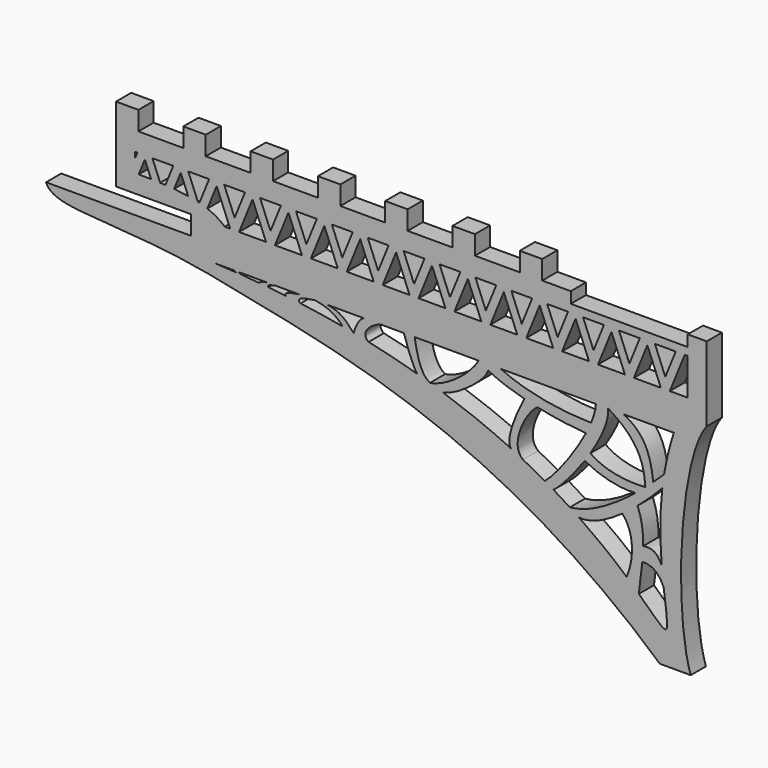
from build123d import *

# Parameters (mm, degrees)
F0_W      = 197.5
F0_H      = 25
F1_DEPTH  = 6.35
F2_W      = 7.5
F2_H      = 6.35
F3_DEPTH  = 6.35
F4_DEPTH  = 2.5
F6_DEPTH  = 6.35
F7_W      = 39.1012286186
F7_H      = 3.7313760072
F8_DEPTH  = 25
F9_DEPTH  = 6.3499999233
F5_W      = 6.35
F5_H      = 6.35
F10_DEPTH = 25


# Not quite as in the source:
# - a length typed as a fraction of an inch, garbled in the dataset ("3 / 203.2 mm" for 3/8 in), is restored
# - a feature names something its author has since deleted; it is built from what else it names


with BuildPart() as f1:
    # F0 (on Front) → F1 (new body)
    with BuildSketch(Plane.XZ):
        with BuildLine():
            add(Edge.make_bspline(
                [(98.75, -5), (89.6041318774, -16.6829489172), (87.6455754042, -62.8589260578), (93.393959105, -80)],
                knots=[0, 0, 0, 0, 75.1910046087, 75.1910046087, 75.1910046087, 75.1910046087], degree=3))
            Line((98.75, -5), (-98.75, -5))
            add(Edge.make_bspline(
                [(-98.75, -5), (-63.6426135898, -22.327804938), (7.773979567, -13.3445840329), (83.1019603317, -80)],
                knots=[0, 0, 0, 0, 196.7107914591, 196.7107914591, 196.7107914591, 196.7107914591], degree=3))
            Line((83.1019603317, -80), (93.393959105, -80))
        make_face()
        with BuildLine():
            add(Edge.make_bspline(
                [(-65.759709787, -10.4816574603), (-63.2453230772, -10.5943254224), (-60.7705862807, -10.7313046439), (-58.3349275577, -10.8914524019)],
                knots=[0, 0, 0, 0, 0.0133310218, 0.0133310218, 0.0133310218, 0.0133310218], degree=3))
            Line((-65.759709787, -10.4816574603), (-58.7879791856, -10.4816574603))
            Line((-58.7879791856, -10.4816574603), (-57.3127828538, -10.4816574603))
            Line((-57.3127828538, -10.4816574603), (-47.9639396071, -10.4816574603))
            Line((-47.9639396071, -10.4816574603), (-45.4429499805, -10.4816574603))
            Line((-45.4429499805, -10.4816574603), (-37.5518873334, -10.4816574603))
            Line((-37.5518873334, -10.4816574603), (-32.1224816144, -10.4816574603))
            Line((-32.1224816144, -10.4816574603), (-28.0221402645, -10.4816574603))
            Line((-28.0221402645, -10.4816574603), (-15.9640572965, -10.4816574603))
            Line((-15.9640572965, -10.4816574603), (-10.2372542024, -10.4816574603))
            Line((-10.2372542024, -10.4816574603), (-2.4892275687, -10.4816574603))
            Line((-2.4892275687, -10.4816574603), (1.1040605605, -10.4816574603))
            Line((1.1040605605, -10.4816574603), (22.4099401385, -10.4816574603))
            Line((22.4099401385, -10.4816574603), (29.8736523837, -10.4816574603))
            Line((29.8736523837, -10.4816574603), (61.6671070457, -10.4816574603))
            Line((61.6671070457, -10.4816574603), (65.7978504896, -10.4816574603))
            Line((65.7978504896, -10.4816574603), (70.9762573242, -10.4816574603))
            Line((70.9762573242, -10.4816574603), (87.7543787006, -10.4816574603))
            add(Edge.make_bspline(
                [(84.48485297, -23.7784693837), (85.1953370139, -19.4532237111), (86.2479291527, -14.9932687844), (87.7543787006, -10.4816574603)],
                knots=[0.9407477342, 0.9407477342, 0.9407477342, 0.9407477342, 1, 1, 1, 1], degree=3))
            add(Edge.make_bspline(
                [(83.8869246499, -28.033053302), (84.0513440433, -26.6316839804), (84.2492959554, -25.212480417), (84.48485297, -23.7784693837)],
                knots=[0.9211029766, 0.9211029766, 0.9211029766, 0.9211029766, 0.9407477342, 0.9407477342, 0.9407477342, 0.9407477342], degree=3))
            add(Edge.make_bspline(
                [(83.6848718472, -50.8613183266), (83.1253506402, -44.3545057691), (82.8910647479, -36.5209055368), (83.8869246499, -28.033053302)],
                knots=[0.8021180686, 0.8021180686, 0.8021180686, 0.8021180686, 0.9211029766, 0.9211029766, 0.9211029766, 0.9211029766], degree=3))
            add(Edge.make_bspline(
                [(84.3356357543, -57.0348066686), (84.1048122326, -55.149453926), (83.8758889834, -53.0827045495), (83.6848718472, -50.8613183266)],
                knots=[0.7614973449, 0.7614973449, 0.7614973449, 0.7614973449, 0.8021180686, 0.8021180686, 0.8021180686, 0.8021180686], degree=3))
            add(Edge.make_bspline(
                [(76.0466038547, -61.7151507236), (81.9550720838, -67.2257504262), (86.8926623373, -72.9460572696), (85.1127651831, -63.38235344), (84.3356357543, -57.0348066686)],
                knots=[0.4567156472, 0.4567156472, 0.4567156472, 0.4567156472, 0.62473676, 0.7614973449, 0.7614973449, 0.7614973449, 0.7614973449], degree=3))
            add(Edge.make_bspline(
                [(71.9460187023, -58.0001276881), (73.4569449838, -59.326355576), (74.8203953797, -60.5715135243), (76.0466038547, -61.7151507236)],
                knots=[0.4218455413, 0.4218455413, 0.4218455413, 0.4218455413, 0.4567156472, 0.4567156472, 0.4567156472, 0.4567156472], degree=3))
            add(Edge.make_bspline(
                [(56.0711816028, -45.7453459696), (62.6000337954, -50.1569782108), (67.8222936938, -54.380494371), (71.9460187023, -58.0001276881)],
                knots=[0.3266756252, 0.3266756252, 0.3266756252, 0.3266756252, 0.4218455413, 0.4218455413, 0.4218455413, 0.4218455413], degree=3))
            add(Edge.make_bspline(
                [(53.0046953922, -43.7233264114), (54.0574936691, -44.4007021836), (55.0794126404, -45.0751944941), (56.0711816028, -45.7453459696)],
                knots=[0.3122187856, 0.3122187856, 0.3122187856, 0.3122187856, 0.3266756252, 0.3266756252, 0.3266756252, 0.3266756252], degree=3))
            add(Edge.make_bspline(
                [(47.5318004772, -40.3497342585), (49.4425367571, -41.4777534857), (51.2657395603, -42.6044733744), (53.0046953922, -43.7233264114)],
                knots=[0.2883397519, 0.2883397519, 0.2883397519, 0.2883397519, 0.3122187856, 0.3122187856, 0.3122187856, 0.3122187856], degree=3))
            add(Edge.make_bspline(
                [(44.6505962547, -38.6863100754), (45.6324034122, -39.2405788357), (46.5926747482, -39.7953134888), (47.5318004772, -40.3497342585)],
                knots=[0.2766032212, 0.2766032212, 0.2766032212, 0.2766032212, 0.2883397519, 0.2883397519, 0.2883397519, 0.2883397519], degree=3))
            add(Edge.make_bspline(
                [(37.3149573755, -34.7702959798), (39.8841702832, -36.066140887), (42.3276605214, -37.3749214801), (44.6505962547, -38.6863100754)],
                knots=[0.2488348287, 0.2488348287, 0.2488348287, 0.2488348287, 0.2766032212, 0.2766032212, 0.2766032212, 0.2766032212], degree=3))
            add(Edge.make_bspline(
                [(33.3332120345, -32.821860666), (34.6928471757, -33.4671703542), (36.0198749712, -34.1170897262), (37.3149573755, -34.7702959798)],
                knots=[0.234837407, 0.234837407, 0.234837407, 0.234837407, 0.2488348287, 0.2488348287, 0.2488348287, 0.2488348287], degree=3))
            add(Edge.make_bspline(
                [(10.4947332364, -23.681362128), (18.9719825925, -26.5045688693), (26.557499928, -29.605973893), (33.3332120345, -32.821860666)],
                knots=[0.165081561, 0.165081561, 0.165081561, 0.165081561, 0.234837407, 0.234837407, 0.234837407, 0.234837407], degree=3))
            add(Edge.make_bspline(
                [(6.2234793397, -22.3067678937), (7.6717739992, -22.7568947859), (9.0954024691, -23.2153383165), (10.4947332364, -23.681362128)],
                knots=[0.1535670358, 0.1535670358, 0.1535670358, 0.1535670358, 0.165081561, 0.165081561, 0.165081561, 0.165081561], degree=3))
            add(Edge.make_bspline(
                [(1.8814823178, -21.0044059123), (3.35287305, -21.4300274782), (4.8000887896, -21.8643811457), (6.2234793397, -22.3067678937)],
                knots=[0.1422505082, 0.1422505082, 0.1422505082, 0.1422505082, 0.1535670358, 0.1535670358, 0.1535670358, 0.1535670358], degree=3))
            add(Edge.make_bspline(
                [(-14.2821822906, -16.9273048212), (-8.5949395005, -18.1623744753), (-3.2118878299, -19.531073146), (1.8814823178, -21.0044059123)],
                knots=[0.1030771858, 0.1030771858, 0.1030771858, 0.1030771858, 0.1422505082, 0.1422505082, 0.1422505082, 0.1422505082], degree=3))
            add(Edge.make_bspline(
                [(-19.2551519245, -15.8974694935), (-17.5722033157, -16.2292806482), (-15.9146611567, -16.5727876707), (-14.2821822906, -16.9273048212)],
                knots=[0.0918327879, 0.0918327879, 0.0918327879, 0.0918327879, 0.1030771858, 0.1030771858, 0.1030771858, 0.1030771858], degree=3))
            add(Edge.make_bspline(
                [(-22.99176564, -15.187903168), (-21.7325254655, -15.4179794431), (-20.4870324208, -15.6545911977), (-19.2551519245, -15.8974694935)],
                knots=[0.0836021417, 0.0836021417, 0.0836021417, 0.0836021417, 0.0918327879, 0.0918327879, 0.0918327879, 0.0918327879], degree=3))
            add(Edge.make_bspline(
                [(-37.0301090074, -12.9832383793), (-32.170871054, -13.6264103929), (-27.4934728723, -14.365394442), (-22.99176564, -15.187903168)],
                knots=[0.0541780811, 0.0541780811, 0.0541780811, 0.0541780811, 0.0836021417, 0.0836021417, 0.0836021417, 0.0836021417], degree=3))
            add(Edge.make_bspline(
                [(-41.8800378972, -12.3806058964), (-40.2436101899, -12.5708446493), (-38.6270399752, -12.7718675191), (-37.0301090074, -12.9832383793)],
                knots=[0.0445082122, 0.0445082122, 0.0445082122, 0.0445082122, 0.0541780811, 0.0541780811, 0.0541780811, 0.0541780811], degree=3))
            add(Edge.make_bspline(
                [(-47.8362962746, -11.7451335191), (-45.8222313414, -11.9410389088), (-43.8369362876, -12.1531116371), (-41.8800378972, -12.3806058964)],
                knots=[0.0329446395, 0.0329446395, 0.0329446395, 0.0329446395, 0.0445082122, 0.0445082122, 0.0445082122, 0.0445082122], degree=3))
            add(Edge.make_bspline(
                [(-50.9760160676, -11.4549833836), (-49.9217537521, -11.5473301551), (-48.875197562, -11.6440809868), (-47.8362962746, -11.7451335191)],
                knots=[0.0269798812, 0.0269798812, 0.0269798812, 0.0269798812, 0.0329446395, 0.0329446395, 0.0329446395, 0.0329446395], degree=3))
            add(Edge.make_bspline(
                [(-55.2391494684, -11.108963422), (-53.8042929939, -11.2162939437), (-52.3832891368, -11.3317150824), (-50.9760160676, -11.4549833836)],
                knots=[0.0190178744, 0.0190178744, 0.0190178744, 0.0190178744, 0.0269798812, 0.0269798812, 0.0269798812, 0.0269798812], degree=3))
            add(Edge.make_bspline(
                [(-58.3349275577, -10.8914524019), (-57.2959050051, -10.9597694986), (-56.2639937725, -11.0323027415), (-55.2391494684, -11.108963422)],
                knots=[0.0133310218, 0.0133310218, 0.0133310218, 0.0133310218, 0.0190178744, 0.0190178744, 0.0190178744, 0.0190178744], degree=3))
        make_face(mode=Mode.SUBTRACT)
        with Locations((0, 7.5)):
            Rectangle(F0_W, F0_H)
        Polygon((92.4, 13.65), (92.4, 1.35), (86.4, 1.35), (83.4, 1.35), (74.4, 1.35), (71.4, 1.35), (62.4, 1.35), (59.4, 1.35), (50.4, 1.35), (47.4, 1.35), (38.4, 1.35), (35.4, 1.35), (26.4, 1.35), (23.4, 1.35), (14.4, 1.35), (11.4, 1.35), (2.4, 1.35), (-0.6, 1.35), (-9.6, 1.35), (-12.6, 1.35), (-21.6, 1.35), (-24.6, 1.35), (-33.6, 1.35), (-36.6, 1.35), (-45.6, 1.35), (-48.6, 1.35), (-57.6, 1.35), (-60.6, 1.35), (-62.4, 1.35), (-69.6, 1.35), (-72.6, 1.35), (-81.6, 1.35), (-84.6, 1.35), (-92.4, 1.35), (-92.4, 4.31), (-92.4, 7.35), (-92.4, 11.71), (-92.4, 13.65), (-91.6135135135, 13.65), (-90.6, 16.15), (-89.5864864865, 13.65), (-88.6135135135, 13.65), (-87.6, 16.15), (-86.5864864865, 13.65), (-79.6135135135, 13.65), (-78.6, 16.15), (-77.5864864865, 13.65), (-76.6135135135, 13.65), (-75.6, 16.15), (-74.5864864865, 13.65), (-67.6135135135, 13.65), (-66.6, 16.15), (-65.5864864865, 13.65), (-64.6135135135, 13.65), (-63.6, 16.15), (-62.5864864865, 13.65), (-55.6135135135, 13.65), (-54.6, 16.15), (-53.5864864865, 13.65), (-52.6135135135, 13.65), (-51.6, 16.15), (-50.5864864865, 13.65), (-43.6135135135, 13.65), (-42.6, 16.15), (-41.5864864865, 13.65), (-40.6135135135, 13.65), (-39.6, 16.15), (-38.5864864865, 13.65), (-31.6135135135, 13.65), (-30.6, 16.15), (-29.5864864865, 13.65), (-28.6135135135, 13.65), (-27.6, 16.15), (-26.5864864865, 13.65), (-19.6135135135, 13.65), (-18.6, 16.15), (-17.5864864865, 13.65), (-16.6135135135, 13.65), (-15.6, 16.15), (-14.5864864865, 13.65), (-7.6135135135, 13.65), (-6.6, 16.15), (-5.5864864865, 13.65), (-4.6135135135, 13.65), (-3.6, 16.15), (-2.5864864865, 13.65), (4.3864864865, 13.65), (5.4, 16.15), (6.4135135135, 13.65), (7.3864864865, 13.65), (8.4, 16.15), (9.4135135135, 13.65), (16.3864864865, 13.65), (17.4, 16.15), (18.4135135135, 13.65), (19.3864864865, 13.65), (20.4, 16.15), (21.4135135135, 13.65), (28.3864864865, 13.65), (29.4, 16.15), (30.4135135135, 13.65), (31.3864864865, 13.65), (32.4, 16.15), (33.4135135135, 13.65), (40.3864864865, 13.65), (41.4, 16.15), (42.4135135135, 13.65), (43.3864864865, 13.65), (44.4, 16.15), (45.4135135135, 13.65), (52.3864864865, 13.65), (53.4, 16.15), (54.4135135135, 13.65), (55.3864864865, 13.65), (56.4, 16.15), (57.4135135135, 13.65), (64.3864864865, 13.65), (65.4, 16.15), (66.4135135135, 13.65), (67.3864864865, 13.65), (68.4, 16.15), (69.4135135135, 13.65), (76.3864864865, 13.65), (77.4, 16.15), (78.4135135135, 13.65), (79.3864864865, 13.65), (80.4, 16.15), (81.4135135135, 13.65), (88.3864864865, 13.65), (91.3864864865, 13.65), align=None, mode=Mode.SUBTRACT)
        with BuildLine():
            Line((65.7978504896, -10.4816574603), (61.6671070457, -10.4816574603))
            add(Edge.make_bspline(
                [(60.0847187439, -16.5496386622), (61.0756793988, -14.2032740615), (61.6736950942, -12.0951756308), (61.6671070457, -10.4816574603)],
                knots=[25.462285853, 25.462285853, 25.462285853, 25.462285853, 32.9403106943, 32.9403106943, 32.9403106943, 32.9403106943], degree=3))
            add(Edge.make_bspline(
                [(58.3588024867, -20.1612836249), (59.0126430275, -18.9199905731), (59.5963911144, -17.7058850356), (60.0847187439, -16.5496386622)],
                knots=[21.7772493925, 21.7772493925, 21.7772493925, 21.7772493925, 25.462285853, 25.462285853, 25.462285853, 25.462285853], degree=3))
            add(Edge.make_bspline(
                [(44.6505962547, -38.6863100754), (48.1829739645, -35.7819743058), (54.4948384056, -27.4968822406), (58.3588024867, -20.1612836249)],
                knots=[0, 0, 0, 0, 21.7772493925, 21.7772493925, 21.7772493925, 21.7772493925], degree=3))
            add(Edge.make_bspline(
                [(44.6505962547, -38.6863100754), (45.6324034122, -39.2405788357), (46.5926747482, -39.7953134888), (47.5318004772, -40.3497342585)],
                knots=[0.2766032212, 0.2766032212, 0.2766032212, 0.2766032212, 0.2883397519, 0.2883397519, 0.2883397519, 0.2883397519], degree=3))
            add(Edge.make_bspline(
                [(57.9517171021, -28.4242599565), (54.3108044366, -33.6350813387), (50.2093884078, -38.282844387), (47.5318004772, -40.3497342585)],
                knots=[19.2539293083, 19.2539293083, 19.2539293083, 19.2539293083, 35.0107211391, 35.0107211391, 35.0107211391, 35.0107211391], degree=3))
            add(Edge.make_bspline(
                [(59.8575436042, -25.5745284736), (59.2443879934, -26.5348050429), (58.6054762028, -27.4886094167), (57.9517171021, -28.4242599565)],
                knots=[16.4246535187, 16.4246535187, 16.4246535187, 16.4246535187, 19.2539293083, 19.2539293083, 19.2539293083, 19.2539293083], degree=3))
            add(Edge.make_bspline(
                [(65.7978504896, -10.4816574603), (66.1085797514, -14.2071182078), (63.4170652659, -19.9998828383), (59.8575436042, -25.5745284736)],
                knots=[0, 0, 0, 0, 16.4246535187, 16.4246535187, 16.4246535187, 16.4246535187], degree=3))
        make_face()
        with BuildLine():
            Line((29.8736523837, -10.4816574603), (22.4099401385, -10.4816574603))
            add(Edge.make_bspline(
                [(25.6780489338, -12.3534352143), (24.4977620539, -11.7616059964), (23.4022584509, -11.1376377151), (22.4099401385, -10.4816574603)],
                knots=[32.7980602328, 32.7980602328, 32.7980602328, 32.7980602328, 37.2292340348, 37.2292340348, 37.2292340348, 37.2292340348], degree=3))
            add(Edge.make_bspline(
                [(37.7584589003, -16.7207107112), (33.3129817339, -15.5423673153), (29.1324045595, -14.0855468079), (25.6780489338, -12.3534352143)],
                knots=[19.8293062687, 19.8293062687, 19.8293062687, 19.8293062687, 32.7980602328, 32.7980602328, 32.7980602328, 32.7980602328], degree=3))
            add(Edge.make_bspline(
                [(42.1803625343, -17.7854881771), (40.6888661107, -17.4603079049), (39.2095499868, -17.1053451464), (37.7584589003, -16.7207107112)],
                knots=[15.5960501804, 15.5960501804, 15.5960501804, 15.5960501804, 19.8293062687, 19.8293062687, 19.8293062687, 19.8293062687], degree=3))
            add(Edge.make_bspline(
                [(58.3588024867, -20.1612836249), (53.3355507823, -19.7772875995), (47.6752942326, -18.9835087403), (42.1803625343, -17.7854881771)],
                knots=[0, 0, 0, 0, 15.5960501804, 15.5960501804, 15.5960501804, 15.5960501804], degree=3))
            add(Edge.make_bspline(
                [(58.3588024867, -20.1612836249), (59.0126430275, -18.9199905731), (59.5963911144, -17.7058850356), (60.0847187439, -16.5496386622)],
                knots=[21.7772493925, 21.7772493925, 21.7772493925, 21.7772493925, 25.462285853, 25.462285853, 25.462285853, 25.462285853], degree=3))
            add(Edge.make_bspline(
                [(60.0847187439, -16.5496386622), (47.3331118165, -16.3230231964), (36.7021560669, -13.6903477833), (29.8736523837, -10.4816574603)],
                knots=[0, 0, 0, 0, 30.8144272458, 30.8144272458, 30.8144272458, 30.8144272458], degree=3))
        make_face()
        with BuildLine():
            add(Edge.make_bspline(
                [(78.2400502629, -29.5795594501), (79.162668759, -28.7799506841), (80.0339477004, -28.0008363248), (80.84262329, -27.2596680265)],
                knots=[27.3886664947, 27.3886664947, 27.3886664947, 27.3886664947, 30.9554664602, 30.9554664602, 30.9554664602, 30.9554664602], degree=3))
            add(Edge.make_bspline(
                [(74.8700098337, -32.3933389933), (76.0498454996, -31.4460030072), (77.1789047527, -30.4992258728), (78.2400502629, -29.5795594501)],
                knots=[23.2863275706, 23.2863275706, 23.2863275706, 23.2863275706, 27.3886664947, 27.3886664947, 27.3886664947, 27.3886664947], degree=3))
            add(Edge.make_bspline(
                [(53.0046953922, -43.7233264114), (59.8396137806, -43.1661743955), (68.1728450446, -37.7707533169), (74.8700098337, -32.3933389933)],
                knots=[0, 0, 0, 0, 23.2863275706, 23.2863275706, 23.2863275706, 23.2863275706], degree=3))
            add(Edge.make_bspline(
                [(53.0046953922, -43.7233264114), (54.0574936691, -44.4007021836), (55.0794126404, -45.0751944941), (56.0711816028, -45.7453459696)],
                knots=[0.3122187856, 0.3122187856, 0.3122187856, 0.3122187856, 0.3266756252, 0.3266756252, 0.3266756252, 0.3266756252], degree=3))
            add(Edge.make_bspline(
                [(56.0711816028, -45.7453459696), (60.2977500573, -46.1208300554), (65.6205880142, -43.3719518378), (70.5272099637, -39.8740143131)],
                knots=[0, 0, 0, 0, 14.8454914625, 14.8454914625, 14.8454914625, 14.8454914625], degree=3))
            add(Edge.make_bspline(
                [(70.5272099637, -39.8740143131), (72.30613066, -38.6058193063), (74.0303413505, -37.2391633124), (75.6277622982, -35.8872449137)],
                knots=[14.8454914625, 14.8454914625, 14.8454914625, 14.8454914625, 20.2277997552, 20.2277997552, 20.2277997552, 20.2277997552], degree=3))
            add(Edge.make_bspline(
                [(75.6277622982, -35.8872449137), (79.4114234149, -32.68508265), (82.4837566461, -29.5656026462), (83.8869246499, -28.033053302)],
                knots=[20.2277997552, 20.2277997552, 20.2277997552, 20.2277997552, 32.9763683993, 32.9763683993, 32.9763683993, 32.9763683993], degree=3))
            add(Edge.make_bspline(
                [(83.8869246499, -28.033053302), (84.0513440433, -26.6316839804), (84.2492959554, -25.212480417), (84.48485297, -23.7784693837)],
                knots=[0.9211029766, 0.9211029766, 0.9211029766, 0.9211029766, 0.9407477342, 0.9407477342, 0.9407477342, 0.9407477342], degree=3))
            add(Edge.make_bspline(
                [(80.84262329, -27.2596680265), (82.2734968467, -25.9482421187), (83.5083724964, -24.7556173344), (84.48485297, -23.7784693837)],
                knots=[30.9554664602, 30.9554664602, 30.9554664602, 30.9554664602, 37.2665754125, 37.2665754125, 37.2665754125, 37.2665754125], degree=3))
        make_face()
        with BuildLine():
            add(Edge.make_bspline(
                [(70.5272099637, -39.8740143131), (74.9861299992, -44.78995502), (74.1921216249, -53.1270802021), (71.9460187023, -58.0001276881)],
                knots=[0, 0, 0, 0, 18.1815567078, 18.1815567078, 18.1815567078, 18.1815567078], degree=3))
            add(Edge.make_bspline(
                [(71.9460187023, -58.0001276881), (73.4569449838, -59.326355576), (74.8203953797, -60.5715135243), (76.0466038547, -61.7151507236)],
                knots=[0.4218455413, 0.4218455413, 0.4218455413, 0.4218455413, 0.4567156472, 0.4567156472, 0.4567156472, 0.4567156472], degree=3))
            add(Edge.make_bspline(
                [(77.2107662738, -51.8775882795), (76.8736521354, -55.2196716314), (76.3424581234, -58.5197961174), (76.0466038547, -61.7151507236)],
                knots=[15.8511875894, 15.8511875894, 15.8511875894, 15.8511875894, 25.8313016856, 25.8313016856, 25.8313016856, 25.8313016856], degree=3))
            add(Edge.make_bspline(
                [(77.5129660357, -47.1400606018), (77.4849713904, -48.7241622392), (77.3693402282, -50.3055172421), (77.2107662738, -51.8775882795)],
                knots=[11.1566762117, 11.1566762117, 11.1566762117, 11.1566762117, 15.8511875894, 15.8511875894, 15.8511875894, 15.8511875894], degree=3))
            add(Edge.make_bspline(
                [(75.6277622982, -35.8872449137), (77.1510621988, -39.5951980588), (77.5794963236, -43.3753857223), (77.5129660357, -47.1400606018)],
                knots=[0, 0, 0, 0, 11.1566762117, 11.1566762117, 11.1566762117, 11.1566762117], degree=3))
            add(Edge.make_bspline(
                [(70.5272099637, -39.8740143131), (72.30613066, -38.6058193063), (74.0303413505, -37.2391633124), (75.6277622982, -35.8872449137)],
                knots=[14.8454914625, 14.8454914625, 14.8454914625, 14.8454914625, 20.2277997552, 20.2277997552, 20.2277997552, 20.2277997552], degree=3))
        make_face()
        with BuildLine():
            Line((70.9762573242, -10.4816574603), (65.7978504896, -10.4816574603))
            add(Edge.make_bspline(
                [(78.2400502629, -29.5795594501), (77.7780916973, -21.8921517618), (75.1671940088, -16.122511588), (65.7978504896, -10.4816574603)],
                knots=[0, 0, 0, 0, 22.7933805217, 22.7933805217, 22.7933805217, 22.7933805217], degree=3))
            add(Edge.make_bspline(
                [(78.2400502629, -29.5795594501), (79.162668759, -28.7799506841), (80.0339477004, -28.0008363248), (80.84262329, -27.2596680265)],
                knots=[27.3886664947, 27.3886664947, 27.3886664947, 27.3886664947, 30.9554664602, 30.9554664602, 30.9554664602, 30.9554664602], degree=3))
            add(Edge.make_bspline(
                [(80.84262329, -27.2596680265), (80.1640096856, -20.6172912009), (78.5020440817, -14.1374813393), (70.9762573242, -10.4816574603)],
                knots=[0, 0, 0, 0, 19.4639876677, 19.4639876677, 19.4639876677, 19.4639876677], degree=3))
        make_face()
        with BuildLine():
            add(Edge.make_bspline(
                [(22.4099401385, -10.4816574603), (20.5344334245, -14.4370757043), (12.4321363532, -21.3281778624), (6.2234793397, -22.3067678937)],
                knots=[0, 0, 0, 0, 20.0458162705, 20.0458162705, 20.0458162705, 20.0458162705], degree=3))
            add(Edge.make_bspline(
                [(6.2234793397, -22.3067678937), (7.6717739992, -22.7568947859), (9.0954024691, -23.2153383165), (10.4947332364, -23.681362128)],
                knots=[0.1535670358, 0.1535670358, 0.1535670358, 0.1535670358, 0.165081561, 0.165081561, 0.165081561, 0.165081561], degree=3))
            add(Edge.make_bspline(
                [(25.6780489338, -12.3534352143), (24.5176322607, -16.0640382603), (15.1727138842, -23.0167808315), (10.4947332364, -23.681362128)],
                knots=[0, 0, 0, 0, 18.9434686298, 18.9434686298, 18.9434686298, 18.9434686298], degree=3))
            add(Edge.make_bspline(
                [(25.6780489338, -12.3534352143), (24.4977620539, -11.7616059964), (23.4022584509, -11.1376377151), (22.4099401385, -10.4816574603)],
                knots=[32.7980602328, 32.7980602328, 32.7980602328, 32.7980602328, 37.2292340348, 37.2292340348, 37.2292340348, 37.2292340348], degree=3))
        make_face()
        with BuildLine():
            add(Edge.make_bspline(
                [(74.8700098337, -32.3933389933), (76.0498454996, -31.4460030072), (77.1789047527, -30.4992258728), (78.2400502629, -29.5795594501)],
                knots=[23.2863275706, 23.2863275706, 23.2863275706, 23.2863275706, 27.3886664947, 27.3886664947, 27.3886664947, 27.3886664947], degree=3))
            add(Edge.make_bspline(
                [(59.8575436042, -25.5745284736), (64.3577575684, -28.8347955793), (71.3215619326, -30.0623122603), (78.2400502629, -29.5795594501)],
                knots=[0, 0, 0, 0, 18.8137403027, 18.8137403027, 18.8137403027, 18.8137403027], degree=3))
            add(Edge.make_bspline(
                [(59.8575436042, -25.5745284736), (59.2443879934, -26.5348050429), (58.6054762028, -27.4886094167), (57.9517171021, -28.4242599565)],
                knots=[16.4246535187, 16.4246535187, 16.4246535187, 16.4246535187, 19.2539293083, 19.2539293083, 19.2539293083, 19.2539293083], degree=3))
            add(Edge.make_bspline(
                [(57.9517171021, -28.4242599565), (61.9971491396, -30.5344350636), (68.0639222264, -32.7770151198), (74.8700098337, -32.3933389933)],
                knots=[0, 0, 0, 0, 17.3776355513, 17.3776355513, 17.3776355513, 17.3776355513], degree=3))
        make_face()
        with BuildLine():
            add(Edge.make_bspline(
                [(37.7584589003, -16.7207107112), (36.0090921977, -19.8501714013), (31.0873150466, -30.4321467039), (33.3332120345, -32.821860666)],
                knots=[0, 0, 0, 0, 16.698198696, 16.698198696, 16.698198696, 16.698198696], degree=3))
            add(Edge.make_bspline(
                [(33.3332120345, -32.821860666), (34.6928471757, -33.4671703542), (36.0198749712, -34.1170897262), (37.3149573755, -34.7702959798)],
                knots=[0.234837407, 0.234837407, 0.234837407, 0.234837407, 0.2488348287, 0.2488348287, 0.2488348287, 0.2488348287], degree=3))
            add(Edge.make_bspline(
                [(42.1803625343, -17.7854881771), (38.6197759533, -20.0084939689), (32.4902777722, -31.0945309624), (37.3149573755, -34.7702959798)],
                knots=[0, 0, 0, 0, 17.667933197, 17.667933197, 17.667933197, 17.667933197], degree=3))
            add(Edge.make_bspline(
                [(42.1803625343, -17.7854881771), (40.6888661107, -17.4603079049), (39.2095499868, -17.1053451464), (37.7584589003, -16.7207107112)],
                knots=[15.5960501804, 15.5960501804, 15.5960501804, 15.5960501804, 19.8293062687, 19.8293062687, 19.8293062687, 19.8293062687], degree=3))
        make_face()
        with BuildLine():
            Line((-92.4, 1.35), (-84.6, 1.35))
            Line((-84.6, 1.35), (-87.0299326713, 7.3438339226))
            add(Edge.make_bspline(
                [(-91.1623099358, 7.362968825), (-89.7087542708, 7.3735352095), (-88.3329530456, 7.3667226405), (-87.0299326713, 7.3438339226)],
                knots=[0.6111811792, 0.6111811792, 0.6111811792, 0.6111811792, 2.7969142011, 2.7969142011, 2.7969142011, 2.7969142011], degree=3))
            Line((-91.1623099358, 7.362968825), (-92.4, 4.31))
            Line((-92.4, 4.31), (-92.4, 1.35))
        make_face()
        with BuildLine():
            Line((-81.6, 1.35), (-72.6, 1.35))
            Line((-72.6, 1.35), (-74.6445363191, 6.3931895871))
            add(Edge.make_bspline(
                [(-79.3242019839, 6.9636351063), (-77.5879288026, 6.8107230955), (-76.0366566301, 6.6183175745), (-74.6445363191, 6.3931895871)],
                knots=[7.685023711, 7.685023711, 7.685023711, 7.685023711, 11.4710988351, 11.4710988351, 11.4710988351, 11.4710988351], degree=3))
            Line((-79.3242019839, 6.9636351063), (-81.6, 1.35))
        make_face()
        with BuildLine():
            add(Edge.make_bspline(
                [(84.3356357543, -57.0348066686), (84.1048122326, -55.149453926), (83.8758889834, -53.0827045495), (83.6848718472, -50.8613183266)],
                knots=[0.7614973449, 0.7614973449, 0.7614973449, 0.7614973449, 0.8021180686, 0.8021180686, 0.8021180686, 0.8021180686], degree=3))
            add(Edge.make_bspline(
                [(77.5129660357, -47.1400606018), (81.1000242829, -46.5764813125), (82.4895426631, -48.2439063489), (83.6848718472, -50.8613183266)],
                knots=[0, 0, 0, 0, 7.2069536144, 7.2069536144, 7.2069536144, 7.2069536144], degree=3))
            add(Edge.make_bspline(
                [(77.5129660357, -47.1400606018), (77.4849713904, -48.7241622392), (77.3693402282, -50.3055172421), (77.2107662738, -51.8775882795)],
                knots=[11.1566762117, 11.1566762117, 11.1566762117, 11.1566762117, 15.8511875894, 15.8511875894, 15.8511875894, 15.8511875894], degree=3))
            add(Edge.make_bspline(
                [(77.2107662738, -51.8775882795), (79.8296034336, -51.8566630781), (82.2116434574, -52.5315739214), (84.3356357543, -57.0348066686)],
                knots=[0, 0, 0, 0, 8.795491267, 8.795491267, 8.795491267, 8.795491267], degree=3))
        make_face()
        with BuildLine():
            Line((1.1040605605, -10.4816574603), (-2.4892275687, -10.4816574603))
            add(Edge.make_bspline(
                [(-2.4892275687, -10.4816574603), (-1.5305990819, -13.7633346021), (0.383801406, -18.9892837864), (1.8814823178, -21.0044059123)],
                knots=[0, 0, 0, 0, 11.3943556156, 11.3943556156, 11.3943556156, 11.3943556156], degree=3))
            add(Edge.make_bspline(
                [(1.8814823178, -21.0044059123), (3.35287305, -21.4300274782), (4.8000887896, -21.8643811457), (6.2234793397, -22.3067678937)],
                knots=[0.1422505082, 0.1422505082, 0.1422505082, 0.1422505082, 0.1535670358, 0.1535670358, 0.1535670358, 0.1535670358], degree=3))
            add(Edge.make_bspline(
                [(6.2234793397, -22.3067678937), (2.6628852488, -20.4860014846), (1.6135276528, -13.426464051), (1.1040605605, -10.4816574603)],
                knots=[0, 0, 0, 0, 12.8857163324, 12.8857163324, 12.8857163324, 12.8857163324], degree=3))
        make_face()
        with BuildLine():
            Line((-10.2372542024, -10.4816574603), (-15.9640572965, -10.4816574603))
            add(Edge.make_bspline(
                [(-15.9640572965, -10.4816574603), (-17.7565403283, -11.405239813), (-19.0194105432, -14.6001277884), (-19.2551519245, -15.8974694935)],
                knots=[0, 0, 0, 0, 6.3373751529, 6.3373751529, 6.3373751529, 6.3373751529], degree=3))
            add(Edge.make_bspline(
                [(-19.2551519245, -15.8974694935), (-17.5722033157, -16.2292806482), (-15.9146611567, -16.5727876707), (-14.2821822906, -16.9273048212)],
                knots=[0.0918327879, 0.0918327879, 0.0918327879, 0.0918327879, 0.1030771858, 0.1030771858, 0.1030771858, 0.1030771858], degree=3))
            add(Edge.make_bspline(
                [(-10.2372542024, -10.4816574603), (-14.8369930685, -11.9666904211), (-16.7967783765, -15.3098717261), (-14.2821822906, -16.9273048212)],
                knots=[0, 0, 0, 0, 7.6097183351, 7.6097183351, 7.6097183351, 7.6097183351], degree=3))
        make_face()
        with BuildLine():
            Line((-28.0221402645, -10.4816574603), (-32.1224816144, -10.4816574603))
            add(Edge.make_bspline(
                [(-32.1224816144, -10.4816574603), (-26.3739395887, -11.374656111), (-24.0345019539, -13.9484412274), (-22.99176564, -15.187903168)],
                knots=[0, 0, 0, 0, 10.2722306665, 10.2722306665, 10.2722306665, 10.2722306665], degree=3))
            add(Edge.make_bspline(
                [(-22.99176564, -15.187903168), (-21.7325254655, -15.4179794431), (-20.4870324208, -15.6545911977), (-19.2551519245, -15.8974694935)],
                knots=[0.0836021417, 0.0836021417, 0.0836021417, 0.0836021417, 0.0918327879, 0.0918327879, 0.0918327879, 0.0918327879], degree=3))
            add(Edge.make_bspline(
                [(-19.2551519245, -15.8974694935), (-21.3651643768, -14.2235838269), (-22.4346164614, -11.307887733), (-28.0221402645, -10.4816574603)],
                knots=[0, 0, 0, 0, 10.3049068183, 10.3049068183, 10.3049068183, 10.3049068183], degree=3))
        make_face()
        with BuildLine():
            Line((-69.6, 1.35), (-62.4, 1.35))
            add(Edge.make_bspline(
                [(-68.2077429312, 4.784234103), (-65.461468977, 3.7637652405), (-63.7904450742, 2.5496339353), (-62.4, 1.35)],
                knots=[18.7336175286, 18.7336175286, 18.7336175286, 18.7336175286, 30.5941170816, 30.5941170816, 30.5941170816, 30.5941170816], degree=3))
            Line((-68.2077429312, 4.784234103), (-69.6, 1.35))
        make_face()
        with BuildLine():
            Line((-87.0299326713, 7.3438339226), (-84.6, 1.35))
            Line((-84.6, 1.35), (-83.1, 5.05))
            Line((-83.1, 5.05), (-83.9946804025, 7.2568783261))
            add(Edge.make_bspline(
                [(-87.0299326713, 7.3438339226), (-85.9710046553, 7.3252329052), (-84.9601437029, 7.296014627), (-83.9946804025, 7.2568783261)],
                knots=[2.7969142011, 2.7969142011, 2.7969142011, 2.7969142011, 4.573197963, 4.573197963, 4.573197963, 4.573197963], degree=3))
        make_face()
        with BuildLine():
            Line((-83.1, 5.05), (-81.6, 1.35))
            Line((-81.6, 1.35), (-79.3242019839, 6.9636351063))
            add(Edge.make_bspline(
                [(-82.2396503054, 7.1721959134), (-81.2134817801, 7.1144023953), (-80.2429422559, 7.0445477323), (-79.3242019839, 6.9636351063)],
                knots=[5.6816409906, 5.6816409906, 5.6816409906, 5.6816409906, 7.685023711, 7.685023711, 7.685023711, 7.685023711], degree=3))
            Line((-82.2396503054, 7.1721959134), (-83.1, 5.05))
        make_face()
        with BuildLine():
            Line((-32.1224816144, -10.4816574603), (-37.5518873334, -10.4816574603))
            add(Edge.make_bspline(
                [(-37.5518873334, -10.4816574603), (-39.5294241607, -10.7246097177), (-43.3542957133, -11.6059756945), (-41.8800378972, -12.3806058964)],
                knots=[0, 0, 0, 0, 4.7264037562, 4.7264037562, 4.7264037562, 4.7264037562], degree=3))
            add(Edge.make_bspline(
                [(-41.8800378972, -12.3806058964), (-40.2436101899, -12.5708446493), (-38.6270399752, -12.7718675191), (-37.0301090074, -12.9832383793)],
                knots=[0.0445082122, 0.0445082122, 0.0445082122, 0.0445082122, 0.0541780811, 0.0541780811, 0.0541780811, 0.0541780811], degree=3))
            add(Edge.make_bspline(
                [(-32.1224816144, -10.4816574603), (-37.0871126652, -11.0053345561), (-38.6487748038, -12.0604483888), (-37.0301090074, -12.9832383793)],
                knots=[0, 0, 0, 0, 5.5084220719, 5.5084220719, 5.5084220719, 5.5084220719], degree=3))
        make_face()
        with BuildLine():
            Line((-74.6445363191, 6.3931895871), (-72.6, 1.35))
            Line((-72.6, 1.35), (-71.1, 5.05))
            Line((-71.1, 5.05), (-71.3804824815, 5.7418567877))
            add(Edge.make_bspline(
                [(-74.6445363191, 6.3931895871), (-73.4436123593, 6.1989810895), (-72.3611258914, 5.9804212158), (-71.3804824815, 5.7418567877)],
                knots=[11.4710988351, 11.4710988351, 11.4710988351, 11.4710988351, 14.7371874729, 14.7371874729, 14.7371874729, 14.7371874729], degree=3))
        make_face()
        with BuildLine():
            Line((-71.1, 5.05), (-69.6, 1.35))
            Line((-69.6, 1.35), (-68.2077429312, 4.784234103))
            add(Edge.make_bspline(
                [(-70.8713985904, 5.6138834771), (-69.8813559343, 5.3567733844), (-68.9998261767, 5.0785588143), (-68.2077429312, 4.784234103)],
                knots=[15.3127996729, 15.3127996729, 15.3127996729, 15.3127996729, 18.7336175286, 18.7336175286, 18.7336175286, 18.7336175286], degree=3))
            Line((-70.8713985904, 5.6138834771), (-71.1, 5.05))
        make_face()
        Polygon((-84.6, 1.35), (-81.6, 1.35), (-83.1, 5.05), align=None)
        Polygon((-72.6, 1.35), (-69.6, 1.35), (-71.1, 5.05), align=None)
        with BuildLine():
            Line((-45.4429499805, -10.4816574603), (-47.9639396071, -10.4816574603))
            add(Edge.make_bspline(
                [(-47.9639396071, -10.4816574603), (-49.7504658997, -10.6397052337), (-50.426291577, -11.0352661865), (-50.9760160676, -11.4549833836)],
                knots=[0, 0, 0, 0, 3.1654332968, 3.1654332968, 3.1654332968, 3.1654332968], degree=3))
            add(Edge.make_bspline(
                [(-50.9760160676, -11.4549833836), (-49.9217537521, -11.5473301551), (-48.875197562, -11.6440809868), (-47.8362962746, -11.7451335191)],
                knots=[0.0269798812, 0.0269798812, 0.0269798812, 0.0269798812, 0.0329446395, 0.0329446395, 0.0329446395, 0.0329446395], degree=3))
            add(Edge.make_bspline(
                [(-45.4429499805, -10.4816574603), (-47.6661846042, -10.8779086773), (-48.3162734611, -11.3382417703), (-47.8362962746, -11.7451335191)],
                knots=[0, 0, 0, 0, 2.7063773267, 2.7063773267, 2.7063773267, 2.7063773267], degree=3))
        make_face()
        Polygon((76.3864864865, 13.65), (78.4135135135, 13.65), (77.4, 16.15), align=None)
        Polygon((79.3864864865, 13.65), (81.4135135135, 13.65), (80.4, 16.15), align=None)
        Polygon((-88.6135135135, 13.65), (-86.5864864865, 13.65), (-87.6, 16.15), align=None)
        Polygon((-91.6135135135, 13.65), (-89.5864864865, 13.65), (-90.6, 16.15), align=None)
        Polygon((-79.6135135135, 13.65), (-77.5864864865, 13.65), (-78.6, 16.15), align=None)
        Polygon((-76.6135135135, 13.65), (-74.5864864865, 13.65), (-75.6, 16.15), align=None)
        Polygon((-67.6135135135, 13.65), (-65.5864864865, 13.65), (-66.6, 16.15), align=None)
        Polygon((-64.6135135135, 13.65), (-62.5864864865, 13.65), (-63.6, 16.15), align=None)
        Polygon((-55.6135135135, 13.65), (-53.5864864865, 13.65), (-54.6, 16.15), align=None)
        Polygon((-52.6135135135, 13.65), (-50.5864864865, 13.65), (-51.6, 16.15), align=None)
        Polygon((-43.6135135135, 13.65), (-41.5864864865, 13.65), (-42.6, 16.15), align=None)
        Polygon((-40.6135135135, 13.65), (-38.5864864865, 13.65), (-39.6, 16.15), align=None)
        Polygon((-31.6135135135, 13.65), (-29.5864864865, 13.65), (-30.6, 16.15), align=None)
        Polygon((-28.6135135135, 13.65), (-26.5864864865, 13.65), (-27.6, 16.15), align=None)
        Polygon((-19.6135135135, 13.65), (-17.5864864865, 13.65), (-18.6, 16.15), align=None)
        Polygon((-16.6135135135, 13.65), (-14.5864864865, 13.65), (-15.6, 16.15), align=None)
        Polygon((-7.6135135135, 13.65), (-5.5864864865, 13.65), (-6.6, 16.15), align=None)
        Polygon((-4.6135135135, 13.65), (-2.5864864865, 13.65), (-3.6, 16.15), align=None)
        Polygon((4.3864864865, 13.65), (6.4135135135, 13.65), (5.4, 16.15), align=None)
        Polygon((7.3864864865, 13.65), (9.4135135135, 13.65), (8.4, 16.15), align=None)
        Polygon((16.3864864865, 13.65), (18.4135135135, 13.65), (17.4, 16.15), align=None)
        Polygon((19.3864864865, 13.65), (21.4135135135, 13.65), (20.4, 16.15), align=None)
        Polygon((28.3864864865, 13.65), (30.4135135135, 13.65), (29.4, 16.15), align=None)
        Polygon((31.3864864865, 13.65), (33.4135135135, 13.65), (32.4, 16.15), align=None)
        Polygon((40.3864864865, 13.65), (42.4135135135, 13.65), (41.4, 16.15), align=None)
        Polygon((43.3864864865, 13.65), (45.4135135135, 13.65), (44.4, 16.15), align=None)
        Polygon((52.3864864865, 13.65), (54.4135135135, 13.65), (53.4, 16.15), align=None)
        Polygon((55.3864864865, 13.65), (57.4135135135, 13.65), (56.4, 16.15), align=None)
        Polygon((64.3864864865, 13.65), (66.4135135135, 13.65), (65.4, 16.15), align=None)
        Polygon((67.3864864865, 13.65), (69.4135135135, 13.65), (68.4, 16.15), align=None)
        with BuildLine():
            Line((-83.9946804025, 7.2568783261), (-83.1, 5.05))
            Line((-83.1, 5.05), (-82.2396503054, 7.1721959134))
            add(Edge.make_bspline(
                [(-83.9946804025, 7.2568783261), (-83.3922084964, 7.2324563498), (-82.8074146848, 7.204172241), (-82.2396503054, 7.1721959134)],
                knots=[4.573197963, 4.573197963, 4.573197963, 4.573197963, 5.6816409906, 5.6816409906, 5.6816409906, 5.6816409906], degree=3))
        make_face()
        with BuildLine():
            Line((-92.4, 7.35), (-92.4, 4.31))
            Line((-92.4, 4.31), (-91.1623099358, 7.362968825))
            add(Edge.make_bspline(
                [(-92.4, 7.35), (-91.9812846094, 7.355700774), (-91.5687575012, 7.3600142211), (-91.1623099358, 7.362968825)],
                knots=[0, 0, 0, 0, 0.6111811792, 0.6111811792, 0.6111811792, 0.6111811792], degree=3))
        make_face()
        with BuildLine():
            Line((-57.3127828538, -10.4816574603), (-58.7879791856, -10.4816574603))
            add(Edge.make_bspline(
                [(-58.7879791856, -10.4816574603), (-60.0471496582, -10.5560934171), (-58.8290696876, -10.7652108255), (-58.3349275577, -10.8914524019)],
                knots=[0, 0, 0, 0, 0.6108908836, 0.6108908836, 0.6108908836, 0.6108908836], degree=3))
            add(Edge.make_bspline(
                [(-58.3349275577, -10.8914524019), (-57.2959050051, -10.9597694986), (-56.2639937725, -11.0323027415), (-55.2391494684, -11.108963422)],
                knots=[0.0133310218, 0.0133310218, 0.0133310218, 0.0133310218, 0.0190178744, 0.0190178744, 0.0190178744, 0.0190178744], degree=3))
            add(Edge.make_bspline(
                [(-57.3127828538, -10.4816574603), (-58.2213290036, -10.6957051903), (-57.2956209102, -10.8545350586), (-55.2391494684, -11.108963422)],
                knots=[0, 0, 0, 0, 2.1664413648, 2.1664413648, 2.1664413648, 2.1664413648], degree=3))
        make_face()
        with BuildLine():
            Line((-71.3804824815, 5.7418567877), (-71.1, 5.05))
            Line((-71.1, 5.05), (-70.8713985904, 5.6138834771))
            add(Edge.make_bspline(
                [(-71.3804824815, 5.7418567877), (-71.2076548662, 5.6998124312), (-71.0379905153, 5.6571467294), (-70.8713985904, 5.6138834771)],
                knots=[14.7371874729, 14.7371874729, 14.7371874729, 14.7371874729, 15.3127996729, 15.3127996729, 15.3127996729, 15.3127996729], degree=3))
        make_face()
    extrude(amount=F1_DEPTH)

    # F2 (on face) → F3 (join)
    with BuildSketch(Plane.XY.offset(20)):
        with Locations((-95, -3.175)):
            Rectangle(F2_W, F2_H)
        with Locations((-72.5, -3.175)):
            Rectangle(F2_W, F2_H)
        with Locations((-50, -3.175)):
            Rectangle(F2_W, F2_H)
        with Locations((-27.5, -3.175)):
            Rectangle(F2_W, F2_H)
        with Locations((-5, -3.175)):
            Rectangle(F2_W, F2_H)
        with Locations((17.5, -3.175)):
            Rectangle(F2_W, F2_H)
        with Locations((40, -3.175)):
            Rectangle(F2_W, F2_H)
    extrude(amount=F3_DEPTH)

    # F4 (cut): a face of the model
    f4_faces = [f1.faces().sort_by_distance(p)[0] for p in [
        (0, -3.175, 13.65),
    ]]
    extrude(f4_faces, amount=-F4_DEPTH, mode=Mode.SUBTRACT)

    # F0 (on Front) → F6 (join)
    with BuildSketch(Plane.XZ):
        with Locations((0, 7.5)):
            Rectangle(F0_W, F0_H)
        Polygon((92.4, 13.65), (92.4, 1.35), (86.4, 1.35), (83.4, 1.35), (74.4, 1.35), (71.4, 1.35), (62.4, 1.35), (59.4, 1.35), (50.4, 1.35), (47.4, 1.35), (38.4, 1.35), (35.4, 1.35), (26.4, 1.35), (23.4, 1.35), (14.4, 1.35), (11.4, 1.35), (2.4, 1.35), (-0.6, 1.35), (-9.6, 1.35), (-12.6, 1.35), (-21.6, 1.35), (-24.6, 1.35), (-33.6, 1.35), (-36.6, 1.35), (-45.6, 1.35), (-48.6, 1.35), (-57.6, 1.35), (-60.6, 1.35), (-62.4, 1.35), (-69.6, 1.35), (-72.6, 1.35), (-81.6, 1.35), (-84.6, 1.35), (-92.4, 1.35), (-92.4, 4.31), (-92.4, 7.35), (-92.4, 11.71), (-92.4, 13.65), (-91.6135135135, 13.65), (-90.6, 16.15), (-89.5864864865, 13.65), (-88.6135135135, 13.65), (-87.6, 16.15), (-86.5864864865, 13.65), (-79.6135135135, 13.65), (-78.6, 16.15), (-77.5864864865, 13.65), (-76.6135135135, 13.65), (-75.6, 16.15), (-74.5864864865, 13.65), (-67.6135135135, 13.65), (-66.6, 16.15), (-65.5864864865, 13.65), (-64.6135135135, 13.65), (-63.6, 16.15), (-62.5864864865, 13.65), (-55.6135135135, 13.65), (-54.6, 16.15), (-53.5864864865, 13.65), (-52.6135135135, 13.65), (-51.6, 16.15), (-50.5864864865, 13.65), (-43.6135135135, 13.65), (-42.6, 16.15), (-41.5864864865, 13.65), (-40.6135135135, 13.65), (-39.6, 16.15), (-38.5864864865, 13.65), (-31.6135135135, 13.65), (-30.6, 16.15), (-29.5864864865, 13.65), (-28.6135135135, 13.65), (-27.6, 16.15), (-26.5864864865, 13.65), (-19.6135135135, 13.65), (-18.6, 16.15), (-17.5864864865, 13.65), (-16.6135135135, 13.65), (-15.6, 16.15), (-14.5864864865, 13.65), (-7.6135135135, 13.65), (-6.6, 16.15), (-5.5864864865, 13.65), (-4.6135135135, 13.65), (-3.6, 16.15), (-2.5864864865, 13.65), (4.3864864865, 13.65), (5.4, 16.15), (6.4135135135, 13.65), (7.3864864865, 13.65), (8.4, 16.15), (9.4135135135, 13.65), (16.3864864865, 13.65), (17.4, 16.15), (18.4135135135, 13.65), (19.3864864865, 13.65), (20.4, 16.15), (21.4135135135, 13.65), (28.3864864865, 13.65), (29.4, 16.15), (30.4135135135, 13.65), (31.3864864865, 13.65), (32.4, 16.15), (33.4135135135, 13.65), (40.3864864865, 13.65), (41.4, 16.15), (42.4135135135, 13.65), (43.3864864865, 13.65), (44.4, 16.15), (45.4135135135, 13.65), (52.3864864865, 13.65), (53.4, 16.15), (54.4135135135, 13.65), (55.3864864865, 13.65), (56.4, 16.15), (57.4135135135, 13.65), (64.3864864865, 13.65), (65.4, 16.15), (66.4135135135, 13.65), (67.3864864865, 13.65), (68.4, 16.15), (69.4135135135, 13.65), (76.3864864865, 13.65), (77.4, 16.15), (78.4135135135, 13.65), (79.3864864865, 13.65), (80.4, 16.15), (81.4135135135, 13.65), (88.3864864865, 13.65), (91.3864864865, 13.65), align=None, mode=Mode.SUBTRACT)
        Polygon((84.9, 5.05), (86.4, 1.35), (91.3864864865, 13.65), (88.3864864865, 13.65), align=None)
        Polygon((78.9, 12.45), (83.4, 1.35), (84.9, 5.05), (81.4135135135, 13.65), (79.3864864865, 13.65), align=None)
        Polygon((72.9, 5.05), (74.4, 1.35), (78.9, 12.45), (78.4135135135, 13.65), (76.3864864865, 13.65), align=None)
        Polygon((66.9, 12.45), (71.4, 1.35), (72.9, 5.05), (69.4135135135, 13.65), (67.3864864865, 13.65), align=None)
        Polygon((60.9, 5.05), (62.4, 1.35), (66.9, 12.45), (66.4135135135, 13.65), (64.3864864865, 13.65), align=None)
        Polygon((54.9, 12.45), (59.4, 1.35), (60.9, 5.05), (57.4135135135, 13.65), (55.3864864865, 13.65), align=None)
        Polygon((48.9, 5.05), (50.4, 1.35), (54.9, 12.45), (54.4135135135, 13.65), (52.3864864865, 13.65), align=None)
        Polygon((42.9, 12.45), (47.4, 1.35), (48.9, 5.05), (45.4135135135, 13.65), (43.3864864865, 13.65), align=None)
        Polygon((36.9, 5.05), (38.4, 1.35), (42.9, 12.45), (42.4135135135, 13.65), (40.3864864865, 13.65), align=None)
        Polygon((30.9, 12.45), (35.4, 1.35), (36.9, 5.05), (33.4135135135, 13.65), (31.3864864865, 13.65), align=None)
        Polygon((24.9, 5.05), (26.4, 1.35), (30.9, 12.45), (30.4135135135, 13.65), (28.3864864865, 13.65), align=None)
        Polygon((18.9, 12.45), (23.4, 1.35), (24.9, 5.05), (21.4135135135, 13.65), (19.3864864865, 13.65), align=None)
        Polygon((12.9, 5.05), (14.4, 1.35), (18.9, 12.45), (18.4135135135, 13.65), (16.3864864865, 13.65), align=None)
        Polygon((6.9, 12.45), (11.4, 1.35), (12.9, 5.05), (9.4135135135, 13.65), (7.3864864865, 13.65), align=None)
        Polygon((0.9, 5.05), (2.4, 1.35), (6.9, 12.45), (6.4135135135, 13.65), (4.3864864865, 13.65), align=None)
        Polygon((-5.1, 12.45), (-0.6, 1.35), (0.9, 5.05), (-2.5864864865, 13.65), (-4.6135135135, 13.65), align=None)
        Polygon((-11.1, 5.05), (-9.6, 1.35), (-5.1, 12.45), (-5.5864864865, 13.65), (-7.6135135135, 13.65), align=None)
        Polygon((-17.1, 12.45), (-12.6, 1.35), (-11.1, 5.05), (-14.5864864865, 13.65), (-16.6135135135, 13.65), align=None)
        Polygon((-23.1, 5.05), (-21.6, 1.35), (-17.1, 12.45), (-17.5864864865, 13.65), (-19.6135135135, 13.65), align=None)
        Polygon((-29.1, 12.45), (-24.6, 1.35), (-23.1, 5.05), (-26.5864864865, 13.65), (-28.6135135135, 13.65), align=None)
        Polygon((-35.1, 5.05), (-33.6, 1.35), (-29.1, 12.45), (-29.5864864865, 13.65), (-31.6135135135, 13.65), align=None)
        Polygon((-41.1, 12.45), (-36.6, 1.35), (-35.1, 5.05), (-38.5864864865, 13.65), (-40.6135135135, 13.65), align=None)
        Polygon((-47.1, 5.05), (-45.6, 1.35), (-41.1, 12.45), (-41.5864864865, 13.65), (-43.6135135135, 13.65), align=None)
        Polygon((-59.1, 5.05), (-57.6, 1.35), (-53.1, 12.45), (-53.5864864865, 13.65), (-55.6135135135, 13.65), align=None)
        Polygon((-65.1, 12.45), (-60.6, 1.35), (-59.1, 5.05), (-62.5864864865, 13.65), (-64.6135135135, 13.65), align=None)
        Polygon((-53.1, 12.45), (-48.6, 1.35), (-47.1, 5.05), (-50.5864864865, 13.65), (-52.6135135135, 13.65), align=None)
        with BuildLine():
            Line((-68.2077429312, 4.784234103), (-65.1, 12.45))
            Line((-65.1, 12.45), (-65.5864864865, 13.65))
            Line((-65.5864864865, 13.65), (-67.6135135135, 13.65))
            Line((-67.6135135135, 13.65), (-70.8713985904, 5.6138834771))
            add(Edge.make_bspline(
                [(-70.8713985904, 5.6138834771), (-69.8813559343, 5.3567733844), (-68.9998261767, 5.0785588143), (-68.2077429312, 4.784234103)],
                knots=[15.3127996729, 15.3127996729, 15.3127996729, 15.3127996729, 18.7336175286, 18.7336175286, 18.7336175286, 18.7336175286], degree=3))
        make_face()
        with BuildLine():
            Line((-77.1, 12.45), (-74.6445363191, 6.3931895871))
            add(Edge.make_bspline(
                [(-74.6445363191, 6.3931895871), (-73.4436123593, 6.1989810895), (-72.3611258914, 5.9804212158), (-71.3804824815, 5.7418567877)],
                knots=[11.4710988351, 11.4710988351, 11.4710988351, 11.4710988351, 14.7371874729, 14.7371874729, 14.7371874729, 14.7371874729], degree=3))
            Line((-71.3804824815, 5.7418567877), (-74.5864864865, 13.65))
            Line((-74.5864864865, 13.65), (-76.6135135135, 13.65))
            Line((-76.6135135135, 13.65), (-77.1, 12.45))
        make_face()
        with BuildLine():
            add(Edge.make_bspline(
                [(-82.2396503054, 7.1721959134), (-81.2134817801, 7.1144023953), (-80.2429422559, 7.0445477323), (-79.3242019839, 6.9636351063)],
                knots=[5.6816409906, 5.6816409906, 5.6816409906, 5.6816409906, 7.685023711, 7.685023711, 7.685023711, 7.685023711], degree=3))
            Line((-79.3242019839, 6.9636351063), (-77.1, 12.45))
            Line((-77.1, 12.45), (-77.5864864865, 13.65))
            Line((-77.5864864865, 13.65), (-79.6135135135, 13.65))
            Line((-79.6135135135, 13.65), (-82.2396503054, 7.1721959134))
        make_face()
        with BuildLine():
            Line((-89.1, 12.45), (-87.0299326713, 7.3438339226))
            add(Edge.make_bspline(
                [(-87.0299326713, 7.3438339226), (-85.9710046553, 7.3252329052), (-84.9601437029, 7.296014627), (-83.9946804025, 7.2568783261)],
                knots=[2.7969142011, 2.7969142011, 2.7969142011, 2.7969142011, 4.573197963, 4.573197963, 4.573197963, 4.573197963], degree=3))
            Line((-83.9946804025, 7.2568783261), (-86.5864864865, 13.65))
            Line((-86.5864864865, 13.65), (-88.6135135135, 13.65))
            Line((-88.6135135135, 13.65), (-89.1, 12.45))
        make_face()
        with BuildLine():
            add(Edge.make_bspline(
                [(-92.4, 7.35), (-91.9812846094, 7.355700774), (-91.5687575012, 7.3600142211), (-91.1623099358, 7.362968825)],
                knots=[0, 0, 0, 0, 0.6111811792, 0.6111811792, 0.6111811792, 0.6111811792], degree=3))
            Line((-91.1623099358, 7.362968825), (-89.1, 12.45))
            Line((-89.1, 12.45), (-89.5864864865, 13.65))
            Line((-89.5864864865, 13.65), (-91.6135135135, 13.65))
            Line((-91.6135135135, 13.65), (-92.4, 11.71))
            Line((-92.4, 11.71), (-92.4, 7.35))
        make_face()
        Polygon((71.4, 1.35), (74.4, 1.35), (72.9, 5.05), align=None)
        Polygon((83.4, 1.35), (86.4, 1.35), (84.9, 5.05), align=None)
        Polygon((59.4, 1.35), (62.4, 1.35), (60.9, 5.05), align=None)
        Polygon((47.4, 1.35), (50.4, 1.35), (48.9, 5.05), align=None)
        Polygon((35.4, 1.35), (38.4, 1.35), (36.9, 5.05), align=None)
        Polygon((23.4, 1.35), (26.4, 1.35), (24.9, 5.05), align=None)
        Polygon((11.4, 1.35), (14.4, 1.35), (12.9, 5.05), align=None)
        Polygon((-0.6, 1.35), (2.4, 1.35), (0.9, 5.05), align=None)
        Polygon((-12.6, 1.35), (-9.6, 1.35), (-11.1, 5.05), align=None)
        Polygon((-24.6, 1.35), (-21.6, 1.35), (-23.1, 5.05), align=None)
        Polygon((-36.6, 1.35), (-33.6, 1.35), (-35.1, 5.05), align=None)
        Polygon((-48.6, 1.35), (-45.6, 1.35), (-47.1, 5.05), align=None)
        Polygon((-60.6, 1.35), (-57.6, 1.35), (-59.1, 5.05), align=None)
        Polygon((76.3864864865, 13.65), (78.4135135135, 13.65), (77.4, 16.15), align=None)
        Polygon((79.3864864865, 13.65), (81.4135135135, 13.65), (80.4, 16.15), align=None)
        Polygon((67.3864864865, 13.65), (69.4135135135, 13.65), (68.4, 16.15), align=None)
        Polygon((64.3864864865, 13.65), (66.4135135135, 13.65), (65.4, 16.15), align=None)
        Polygon((55.3864864865, 13.65), (57.4135135135, 13.65), (56.4, 16.15), align=None)
        Polygon((52.3864864865, 13.65), (54.4135135135, 13.65), (53.4, 16.15), align=None)
        Polygon((43.3864864865, 13.65), (45.4135135135, 13.65), (44.4, 16.15), align=None)
        Polygon((40.3864864865, 13.65), (42.4135135135, 13.65), (41.4, 16.15), align=None)
        Polygon((31.3864864865, 13.65), (33.4135135135, 13.65), (32.4, 16.15), align=None)
        Polygon((28.3864864865, 13.65), (30.4135135135, 13.65), (29.4, 16.15), align=None)
        Polygon((19.3864864865, 13.65), (21.4135135135, 13.65), (20.4, 16.15), align=None)
        Polygon((16.3864864865, 13.65), (18.4135135135, 13.65), (17.4, 16.15), align=None)
        Polygon((4.3864864865, 13.65), (6.4135135135, 13.65), (5.4, 16.15), align=None)
        Polygon((7.3864864865, 13.65), (9.4135135135, 13.65), (8.4, 16.15), align=None)
        Polygon((-4.6135135135, 13.65), (-2.5864864865, 13.65), (-3.6, 16.15), align=None)
        Polygon((-7.6135135135, 13.65), (-5.5864864865, 13.65), (-6.6, 16.15), align=None)
        Polygon((-16.6135135135, 13.65), (-14.5864864865, 13.65), (-15.6, 16.15), align=None)
        Polygon((-19.6135135135, 13.65), (-17.5864864865, 13.65), (-18.6, 16.15), align=None)
        Polygon((-28.6135135135, 13.65), (-26.5864864865, 13.65), (-27.6, 16.15), align=None)
        Polygon((-31.6135135135, 13.65), (-29.5864864865, 13.65), (-30.6, 16.15), align=None)
        Polygon((-40.6135135135, 13.65), (-38.5864864865, 13.65), (-39.6, 16.15), align=None)
        Polygon((-43.6135135135, 13.65), (-41.5864864865, 13.65), (-42.6, 16.15), align=None)
        Polygon((-52.6135135135, 13.65), (-50.5864864865, 13.65), (-51.6, 16.15), align=None)
        Polygon((-55.6135135135, 13.65), (-53.5864864865, 13.65), (-54.6, 16.15), align=None)
        Polygon((-64.6135135135, 13.65), (-62.5864864865, 13.65), (-63.6, 16.15), align=None)
        Polygon((-67.6135135135, 13.65), (-65.5864864865, 13.65), (-66.6, 16.15), align=None)
        Polygon((-76.6135135135, 13.65), (-74.5864864865, 13.65), (-75.6, 16.15), align=None)
        Polygon((-79.6135135135, 13.65), (-77.5864864865, 13.65), (-78.6, 16.15), align=None)
        Polygon((-88.6135135135, 13.65), (-86.5864864865, 13.65), (-87.6, 16.15), align=None)
        Polygon((-91.6135135135, 13.65), (-89.5864864865, 13.65), (-90.6, 16.15), align=None)
        Polygon((78.4135135135, 13.65), (78.9, 12.45), (79.3864864865, 13.65), align=None)
        Polygon((54.4135135135, 13.65), (54.9, 12.45), (55.3864864865, 13.65), align=None)
        Polygon((66.4135135135, 13.65), (66.9, 12.45), (67.3864864865, 13.65), align=None)
        Polygon((30.4135135135, 13.65), (30.9, 12.45), (31.3864864865, 13.65), align=None)
        Polygon((18.4135135135, 13.65), (18.9, 12.45), (19.3864864865, 13.65), align=None)
        Polygon((6.4135135135, 13.65), (6.9, 12.45), (7.3864864865, 13.65), align=None)
        Polygon((42.4135135135, 13.65), (42.9, 12.45), (43.3864864865, 13.65), align=None)
        Polygon((-5.5864864865, 13.65), (-5.1, 12.45), (-4.6135135135, 13.65), align=None)
        Polygon((-17.5864864865, 13.65), (-17.1, 12.45), (-16.6135135135, 13.65), align=None)
        Polygon((-29.5864864865, 13.65), (-29.1, 12.45), (-28.6135135135, 13.65), align=None)
        Polygon((-41.5864864865, 13.65), (-41.1, 12.45), (-40.6135135135, 13.65), align=None)
        Polygon((-53.5864864865, 13.65), (-53.1, 12.45), (-52.6135135135, 13.65), align=None)
        Polygon((-65.5864864865, 13.65), (-65.1, 12.45), (-64.6135135135, 13.65), align=None)
        Polygon((-77.5864864865, 13.65), (-77.1, 12.45), (-76.6135135135, 13.65), align=None)
        Polygon((-89.5864864865, 13.65), (-89.1, 12.45), (-88.6135135135, 13.65), align=None)
    extrude(amount=F6_DEPTH)

    # F7 (on face) → F8 (cut)
    with BuildSketch(Plane.XZ.offset(6.35)):
        with Locations((72.8493856907, 18.1343119964)):
            Rectangle(F7_W, F7_H)
    extrude(amount=-F8_DEPTH, mode=Mode.SUBTRACT)

    # F7 (on face) → F9 (join)
    with BuildSketch(Plane.XZ.offset(6.35)):
        with BuildLine():
            add(Edge.make_bspline(
                [(-122.1300065517, -5), (-119.4510546823, -12.2630709037), (-99.3290119272, -8.4670443244), (-67.7505394222, -14.317072571)],
                knots=[0, 0, 0, 0, 55.171861366, 55.171861366, 55.171861366, 55.171861366], degree=3))
            add(Edge.make_bspline(
                [(-98.75, -5), (-90.3483070412, -9.1467882296), (-79.8671406581, -11.786711289), (-67.7505394222, -14.317072571)],
                knots=[0, 0, 0, 0, 47.075668129, 47.075668129, 47.075668129, 47.075668129], degree=3))
            Line((-98.75, -5), (-122.1300065517, -5))
        make_face()
    extrude(amount=-F9_DEPTH)

    # F5 (on face) → F10 (cut)
    with BuildSketch(Plane(origin=(-98.75, 0, 0), x_dir=(0, -1, 0), z_dir=(-1, 0, 0))):
        with Locations((3.175, -1.825)):
            Rectangle(F5_W, F5_H)
    extrude(amount=-F10_DEPTH, mode=Mode.SUBTRACT)


solid = f1.part
